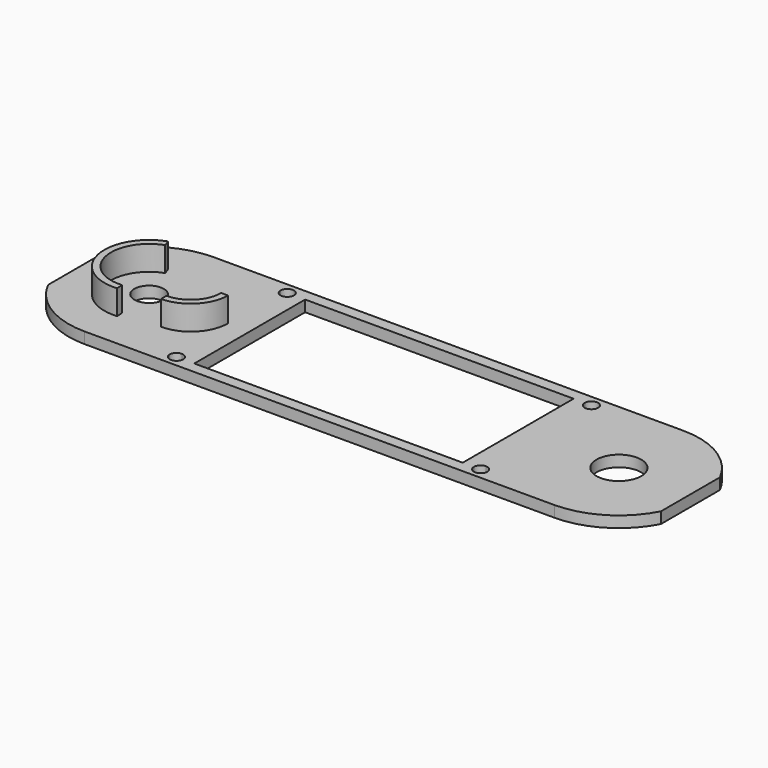
from build123d import *

# Parameters (mm, degrees)
F0_R     = 30
F0_R_2   = 10
F0_R_3   = 14
F0_R_4   = 6.6
F1_DEPTH = 5
F3_DEPTH = 11


with BuildPart() as f1:
    # F0 (on Top) → F1 (new body)
    with BuildSketch(Plane.XY):
        with BuildLine():
            ThreePointArc((18.3030052177, -31), (31.2642622481, -17.8478543831), (36, 0))
            ThreePointArc((36, 0), (31.2978497092, 17.7888898917), (18.4197442455, 30.9307779069))
            ThreePointArc((18.4197442455, 30.9307779069), (9.5522770937, 34.7095664382), (0, 36))
            ThreePointArc((0, 36), (-18.7386337537, 30.7386337537), (-32, 16.4924225025))
            Line((-32, 16.4924225025), (-32, -16.4924225025))
            ThreePointArc((-32, -16.4924225025), (-18.7386337537, -30.7386337537), (0, -36))
            ThreePointArc((0, -36), (9.4868329805, -34.7275107084), (18.3030052177, -31))
        make_face()
        Circle(F0_R, mode=Mode.SUBTRACT)
        with BuildLine():
            ThreePointArc((242, 16.4924225025), (228.7386337537, 30.7386337537), (210, 36))
            ThreePointArc((210, 36), (200.4477229063, 34.7095664382), (191.5802557545, 30.9307779069))
            ThreePointArc((191.5802557545, 30.9307779069), (174.0000639573, -0.0678595955), (191.6969947823, -31))
            ThreePointArc((191.6969947823, -31), (200.5131670195, -34.7275107084), (210, -36))
            ThreePointArc((210, -36), (228.7386337537, -30.7386337537), (242, -16.4924225025))
            Line((242, -16.4924225025), (242, 16.4924225025))
        make_face()
        with Locations((210, 0)):
            Circle(F0_R, mode=Mode.SUBTRACT)
        Circle(F0_R)
        Circle(F0_R_2, mode=Mode.SUBTRACT)
        with Locations((210, 0)):
            Circle(F0_R)
        with Locations((210, 0)):
            Circle(F0_R_3, mode=Mode.SUBTRACT)
        with BuildLine():
            ThreePointArc((19.6214168703, 36), (23.4046464655, 33.6633706545), (26.9125802938, 30.9307779069))
            Line((26.9125802938, 30.9307779069), (34, 30.9307779069))
            ThreePointArc((34, 30.9307779069), (37, 33.9307779069), (40, 30.9307779069))
            Line((40, 30.9307779069), (45, 30.9307779069))
            Line((45, 30.9307779069), (165, 30.9307779069))
            Line((165, 30.9307779069), (170, 30.9307779069))
            ThreePointArc((170, 30.9307779069), (173, 33.9307779069), (176, 30.9307779069))
            Line((176, 30.9307779069), (183.0874197062, 30.9307779069))
            ThreePointArc((183.0874197062, 30.9307779069), (186.5953535345, 33.6633706545), (190.3785831296, 36))
            Line((190.3785831296, 36), (19.6214168703, 36))
        make_face()
        with BuildLine():
            Line((34, -31), (26.83281573, -31))
            ThreePointArc((26.83281573, -31), (23.361269906, -33.693487032), (19.6214168703, -36))
            Line((19.6214168703, -36), (190.3785831296, -36))
            ThreePointArc((190.3785831296, -36), (186.638730094, -33.693487032), (183.16718427, -31))
            Line((183.16718427, -31), (176, -31))
            ThreePointArc((176, -31), (173, -34), (170, -31))
            Line((170, -31), (165, -31))
            Line((165, -31), (45, -31))
            Line((45, -31), (40, -31))
            ThreePointArc((40, -31), (37, -34), (34, -31))
        make_face()
        with Locations((210, 0)):
            Circle(F0_R_3)
        with Locations((210, 0)):
            Circle(F0_R_2, mode=Mode.SUBTRACT)
        with BuildLine():
            Line((37, 27.9307779069), (37, 17.6635217327))
            ThreePointArc((37, 17.6635217327), (39.9874980463, 9.0553851381), (41, 0))
            ThreePointArc((41, 0), (39.9874980463, -9.0553851381), (37, -17.6635217327))
            Line((37, -17.6635217327), (37, -28))
            ThreePointArc((37, -28), (39.1213203436, -28.8786796564), (40, -31))
            Line((40, -31), (45, -31))
            Line((45, -31), (45, 30.9307779069))
            Line((45, 30.9307779069), (40, 30.9307779069))
            ThreePointArc((40, 30.9307779069), (39.1213203436, 28.8094575634), (37, 27.9307779069))
        make_face()
        with BuildLine():
            ThreePointArc((173, -17.6635217327), (169, 0), (173, 17.6635217327))
            Line((173, 17.6635217327), (173, 27.9307779069))
            ThreePointArc((173, 27.9307779069), (170.8786796564, 28.8094575634), (170, 30.9307779069))
            Line((170, 30.9307779069), (165, 30.9307779069))
            Line((165, 30.9307779069), (165, -31))
            Line((165, -31), (170, -31))
            ThreePointArc((170, -31), (170.8786796564, -28.8786796564), (173, -28))
            Line((173, -28), (173, -17.6635217327))
        make_face()
        Circle(F0_R_2)
        Circle(F0_R_4, mode=Mode.SUBTRACT)
        with BuildLine():
            ThreePointArc((18.4197442455, 30.9307779069), (31.2978497092, 17.7888898917), (36, 0))
            ThreePointArc((36, 0), (31.2642622481, -17.8478543831), (18.3030052177, -31))
            Line((18.3030052177, -31), (26.83281573, -31))
            ThreePointArc((26.83281573, -31), (32.6055594055, -24.8571417474), (37, -17.6635217327))
            Line((37, -17.6635217327), (37, 17.6635217327))
            ThreePointArc((37, 17.6635217327), (32.6375474194, 24.815126404), (26.9125802938, 30.9307779069))
            Line((26.9125802938, 30.9307779069), (18.4197442455, 30.9307779069))
        make_face()
        with BuildLine():
            Line((191.5802557545, 30.9307779069), (183.0874197062, 30.9307779069))
            ThreePointArc((183.0874197062, 30.9307779069), (177.3624525806, 24.815126404), (173, 17.6635217327))
            Line((173, 17.6635217327), (173, -17.6635217327))
            ThreePointArc((173, -17.6635217327), (177.3944405945, -24.8571417474), (183.16718427, -31))
            Line((183.16718427, -31), (191.6969947823, -31))
            ThreePointArc((191.6969947823, -31), (174.0000639573, -0.0678595955), (191.5802557545, 30.9307779069))
        make_face()
        with BuildLine():
            ThreePointArc((41, 0), (39.9874980463, 9.0553851381), (37, 17.6635217327))
            Line((37, 17.6635217327), (37, -17.6635217327))
            ThreePointArc((37, -17.6635217327), (39.9874980463, -9.0553851381), (41, 0))
        make_face()
        with BuildLine():
            Line((173, -17.6635217327), (173, 17.6635217327))
            ThreePointArc((173, 17.6635217327), (169, 0), (173, -17.6635217327))
        make_face()
        with BuildLine():
            ThreePointArc((0, 36), (9.5522770937, 34.7095664382), (18.4197442455, 30.9307779069))
            Line((18.4197442455, 30.9307779069), (26.9125802938, 30.9307779069))
            ThreePointArc((26.9125802938, 30.9307779069), (23.4046464655, 33.6633706545), (19.6214168703, 36))
            Line((19.6214168703, 36), (0, 36))
        make_face()
        with BuildLine():
            Line((210, 36), (190.3785831296, 36))
            ThreePointArc((190.3785831296, 36), (186.5953535345, 33.6633706545), (183.0874197062, 30.9307779069))
            Line((183.0874197062, 30.9307779069), (191.5802557545, 30.9307779069))
            ThreePointArc((191.5802557545, 30.9307779069), (200.4477229063, 34.7095664382), (210, 36))
        make_face()
        with BuildLine():
            Line((26.83281573, -31), (18.3030052177, -31))
            ThreePointArc((18.3030052177, -31), (9.4868329805, -34.7275107084), (0, -36))
            Line((0, -36), (19.6214168703, -36))
            ThreePointArc((19.6214168703, -36), (23.361269906, -33.693487032), (26.83281573, -31))
        make_face()
        with BuildLine():
            ThreePointArc((183.16718427, -31), (186.638730094, -33.693487032), (190.3785831296, -36))
            Line((190.3785831296, -36), (210, -36))
            ThreePointArc((210, -36), (200.5131670195, -34.7275107084), (191.6969947823, -31))
            Line((191.6969947823, -31), (183.16718427, -31))
        make_face()
        with BuildLine():
            ThreePointArc((37, -17.6635217327), (32.6055594055, -24.8571417474), (26.83281573, -31))
            Line((26.83281573, -31), (34, -31))
            ThreePointArc((34, -31), (34.8786796564, -28.8786796564), (37, -28))
            Line((37, -28), (37, -17.6635217327))
        make_face()
        with BuildLine():
            Line((176, -31), (183.16718427, -31))
            ThreePointArc((183.16718427, -31), (177.3944405945, -24.8571417474), (173, -17.6635217327))
            Line((173, -17.6635217327), (173, -28))
            ThreePointArc((173, -28), (175.1213203436, -28.8786796564), (176, -31))
        make_face()
        with BuildLine():
            Line((34, 30.9307779069), (26.9125802938, 30.9307779069))
            ThreePointArc((26.9125802938, 30.9307779069), (32.6375474194, 24.815126404), (37, 17.6635217327))
            Line((37, 17.6635217327), (37, 27.9307779069))
            ThreePointArc((37, 27.9307779069), (34.8786796564, 28.8094575634), (34, 30.9307779069))
        make_face()
        with BuildLine():
            ThreePointArc((173, 17.6635217327), (177.3624525806, 24.815126404), (183.0874197062, 30.9307779069))
            Line((183.0874197062, 30.9307779069), (176, 30.9307779069))
            ThreePointArc((176, 30.9307779069), (175.1213203436, 28.8094575634), (173, 27.9307779069))
            Line((173, 27.9307779069), (173, 17.6635217327))
        make_face()
    extrude(amount=F1_DEPTH)

    # F2 (on face) → F3 (join)
    with BuildSketch(Plane.XY.offset(5)):
        with BuildLine():
            ThreePointArc((32.2300370842, 0), (28.249548951, -9.6195118668), (18.6300370842, -13.6))
            Line((18.6300370842, -13.6), (18.6278837067, -16.5999992272))
            ThreePointArc((18.6278837067, -16.5999992272), (30.3708692945, -11.7408322103), (35.2300363114, 0.0021533775))
            Line((35.2300363114, 0.0021533775), (32.2300370842, 0))
        make_face()
        with BuildLine():
            ThreePointArc((1.4010723087, -16.9409777332), (-16.6169103502, -3.544385222), (-5.6333881929, 16.0382252023))
            Line((-5.6333881929, 16.0382252023), (-6.6291181037, 18.8681584073))
            ThreePointArc((-6.6291181037, 18.8681584073), (-19.550908877, -4.1702067977), (1.6467177805, -19.9309038698))
            Line((1.6467177805, -19.9309038698), (1.4010723087, -16.9409777332))
        make_face()
    extrude(amount=F3_DEPTH)


solid = f1.part
